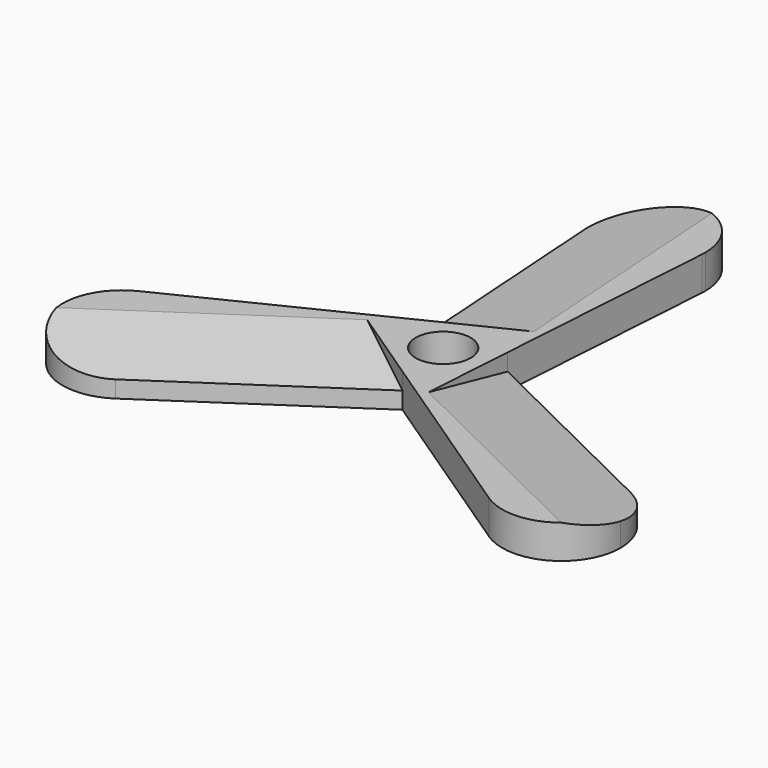
from build123d import *

# Parameters (mm, degrees)
F0_R         = 1.625
F1_DEPTH     = 2
F2_T4_DEPTH  = 23.6841282727
F2_T9_DEPTH  = 23.6841282727
F2_T14_DEPTH = 23.6841282727


# Not quite as in the source:
# - a fillet or chamfer that OpenCascade refuses, or shapes differently, is made with other operations: its cross-section is extruded or revolved along the edge and cut away or added


with BuildPart() as f1:
    # F0 (on Top) → F1 (new body)
    with BuildSketch(Plane.XY):
        with BuildLine():
            ThreePointArc((-3.492213561, 14.7666666667), (0, 11.5), (3.492213561, 14.7666666667))
            ThreePointArc((3.492213561, 14.7666666667), (3.4980528486, 14.8832683922), (3.5, 15))
            ThreePointArc((3.5, 15), (-0.1167316078, 18.4980528486), (-3.492213561, 14.7666666667))
        make_face()
        with BuildLine():
            ThreePointArc((-1.1028815616, 2.2435802328), (0, 2.5), (1.1028815616, 2.2435802328))
            Line((1.1028815616, 2.2435802328), (2.6061068992, 1.5046365198))
            Line((2.6061068992, 1.5046365198), (3.492213561, 14.7666666667))
            ThreePointArc((3.492213561, 14.7666666667), (0, 11.5), (-3.492213561, 14.7666666667))
            Line((-3.492213561, 14.7666666667), (-2.6061068992, 1.5046365198))
            Line((-2.6061068992, 1.5046365198), (-1.1028815616, 2.2435802328))
        make_face()
        with BuildLine():
            Line((2.6061068992, 1.5046365198), (2.4944382578, -0.1666666667))
            ThreePointArc((2.4944382578, -0.1666666667), (2.1650635095, -1.25), (1.3915566962, -2.0769135661))
            Line((1.3915566962, -2.0769135661), (0, -3.0092730395))
            Line((0, -3.0092730395), (11.0422016821, -10.4076789926))
            ThreePointArc((11.0422016821, -10.4076789926), (9.9592921435, -5.75), (14.534415243, -4.3589876741))
            Line((14.534415243, -4.3589876741), (2.6061068992, 1.5046365198))
        make_face()
        with BuildLine():
            ThreePointArc((16.4903810568, -7.5), (15.9614178835, -5.6498810379), (14.534415243, -4.3589876741))
            ThreePointArc((14.534415243, -4.3589876741), (9.9592921435, -5.75), (11.0422016821, -10.4076789926))
            ThreePointArc((11.0422016821, -10.4076789926), (14.6383149433, -10.5877684346), (16.4903810568, -7.5))
        make_face()
        with BuildLine():
            ThreePointArc((-1.3915566962, -2.0769135661), (-2.1650635095, -1.25), (-2.4944382578, -0.1666666667))
            Line((-2.4944382578, -0.1666666667), (-2.6061068992, 1.5046365198))
            Line((-2.6061068992, 1.5046365198), (-14.534415243, -4.3589876741))
            ThreePointArc((-14.534415243, -4.3589876741), (-11.1402620946, -4.5289631732), (-9.4903810568, -7.5))
            ThreePointArc((-9.4903810568, -7.5), (-9.9026126222, -9.1479338865), (-11.0422016821, -10.4076789926))
            Line((-11.0422016821, -10.4076789926), (0, -3.0092730395))
            Line((0, -3.0092730395), (-1.3915566962, -2.0769135661))
        make_face()
        with BuildLine():
            ThreePointArc((-9.4903810568, -7.5), (-11.1402620946, -4.5289631732), (-14.534415243, -4.3589876741))
            ThreePointArc((-14.534415243, -4.3589876741), (-16.02146997, -9.25), (-11.0422016821, -10.4076789926))
            ThreePointArc((-11.0422016821, -10.4076789926), (-9.9026126222, -9.1479338865), (-9.4903810568, -7.5))
        make_face()
        with BuildLine():
            ThreePointArc((1.1028815616, 2.2435802328), (2.122169162, 1.3215135444), (2.5, 0))
            ThreePointArc((2.5, 0), (2.4986091776, -0.0833797199), (2.4944382578, -0.1666666667))
            Line((2.4944382578, -0.1666666667), (2.6061068992, 1.5046365198))
            Line((2.6061068992, 1.5046365198), (1.1028815616, 2.2435802328))
        make_face()
        with BuildLine():
            ThreePointArc((-2.4944382578, -0.1666666667), (-2.1650635095, 1.25), (-1.1028815616, 2.2435802328))
            Line((-1.1028815616, 2.2435802328), (-2.6061068992, 1.5046365198))
            Line((-2.6061068992, 1.5046365198), (-2.4944382578, -0.1666666667))
        make_face()
        with BuildLine():
            Line((0, -3.0092730395), (1.3915566962, -2.0769135661))
            ThreePointArc((1.3915566962, -2.0769135661), (0, -2.5), (-1.3915566962, -2.0769135661))
            Line((-1.3915566962, -2.0769135661), (0, -3.0092730395))
        make_face()
        with BuildLine():
            ThreePointArc((2.4944382578, -0.1666666667), (2.4986091776, -0.0833797199), (2.5, 0))
            ThreePointArc((2.5, 0), (2.122169162, 1.3215135444), (1.1028815616, 2.2435802328))
            ThreePointArc((1.1028815616, 2.2435802328), (0, 2.5), (-1.1028815616, 2.2435802328))
            ThreePointArc((-1.1028815616, 2.2435802328), (-2.1650635095, 1.25), (-2.4944382578, -0.1666666667))
            ThreePointArc((-2.4944382578, -0.1666666667), (-2.1650635095, -1.25), (-1.3915566962, -2.0769135661))
            ThreePointArc((-1.3915566962, -2.0769135661), (0, -2.5), (1.3915566962, -2.0769135661))
            ThreePointArc((1.3915566962, -2.0769135661), (2.1650635095, -1.25), (2.4944382578, -0.1666666667))
        make_face()
        Circle(F0_R, mode=Mode.SUBTRACT)
    extrude(amount=F1_DEPTH)

    # F2: chamfer of 5 x 1 on 3 edges, made by hand


with BuildPart() as f2_tool2:
    # F2_s3 → F2_t4 (new body)
    with BuildSketch(Plane(origin=(-1.3441929146, 20.1180373933, 0), x_dir=(0, 0, 1), z_dir=(0.0666666667, -0.9977753031, 0))):
        with BuildLine():
            Line((0.960776773, 2.6961161351), (2.039223227, -2.6961161351))
            Line((2.039223227, -2.6961161351), (2.139223227, -2.6961161351))
            ThreePointArc((2.139223227, -2.6961161351), (2.1, -0.0980580676), (2.1, 2.5))
            Line((2.1, 2.5), (2, 2.6))
            ThreePointArc((2, 2.6), (1.4803883865, 2.6), (0.960776773, 2.7961161351))
            Line((0.960776773, 2.7961161351), (0.960776773, 2.6961161351))
        make_face()
    extrude(amount=F2_T4_DEPTH)

    split(bisect_by=Plane(origin=(-1.1028815616, 2.2435802328, 0), x_dir=(0, 0, 1), z_dir=(-0.4411526247, 0.8974320931, 0)), keep=Keep.TOP)


with BuildPart() as f1_1:
    add(f1.part)

    # F2_t1: cut F2_tool2
    add(f2_tool2.part, mode=Mode.SUBTRACT)


with BuildPart() as f2_tool7:
    # F2_s8 → F2_t9 (new body)
    with BuildSketch(Plane(origin=(-16.7506349996, -11.2231239083, 0), x_dir=(0, 0, 1), z_dir=(0.8307654265, 0.5566226785, 0))):
        with BuildLine():
            Line((0.960776773, 2.6961161351), (2.039223227, -2.6961161351))
            Line((2.039223227, -2.6961161351), (2.139223227, -2.6961161351))
            ThreePointArc((2.139223227, -2.6961161351), (2.1, -0.0980580676), (2.1, 2.5))
            Line((2.1, 2.5), (2, 2.6))
            ThreePointArc((2, 2.6), (1.4803883865, 2.6), (0.960776773, 2.7961161351))
            Line((0.960776773, 2.7961161351), (0.960776773, 2.6961161351))
        make_face()
    extrude(amount=F2_T9_DEPTH)

    split(bisect_by=Plane(origin=(-1.3915566962, -2.0769135661, 0), x_dir=(0, 0, 1), z_dir=(-0.5566226785, -0.8307654265, 0)), keep=Keep.TOP)


with BuildPart() as f1_2:
    add(f1_1.part)

    # F2_t6: cut F2_tool7
    add(f2_tool7.part, mode=Mode.SUBTRACT)


with BuildPart() as f2_tool12:
    # F2_s13 → F2_t14 (new body)
    with BuildSketch(Plane(origin=(18.0948279142, -8.894913485, 0), x_dir=(0, 0, 1), z_dir=(-0.8974320931, 0.4411526247, 0))):
        with BuildLine():
            Line((0.960776773, 2.6961161351), (2.039223227, -2.6961161351))
            Line((2.039223227, -2.6961161351), (2.139223227, -2.6961161351))
            ThreePointArc((2.139223227, -2.6961161351), (2.1, -0.0980580676), (2.1, 2.5))
            Line((2.1, 2.5), (2, 2.6))
            ThreePointArc((2, 2.6), (1.4803883865, 2.6), (0.960776773, 2.7961161351))
            Line((0.960776773, 2.7961161351), (0.960776773, 2.6961161351))
        make_face()
    extrude(amount=F2_T14_DEPTH)

    split(bisect_by=Plane(origin=(2.4944382578, -0.1666666667, 0), x_dir=(0, 0, 1), z_dir=(0.9977753031, -0.0666666667, 0)), keep=Keep.TOP)


with BuildPart() as f1_3:
    add(f1_2.part)

    # F2_t11: cut F2_tool12
    add(f2_tool12.part, mode=Mode.SUBTRACT)


solid = f1_3.part
